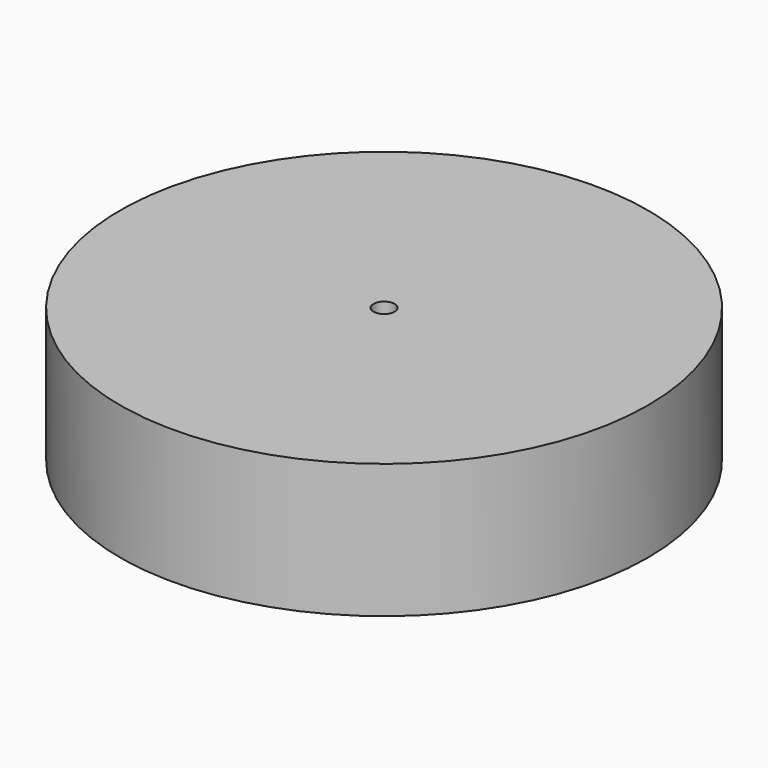
from build123d import *

# Parameters (mm, degrees)
F0_R     = 49.9999
F0_R_2   = 2.0066
F2_DEPTH = 25.4


# Not quite as in the source:
# - the program builds the solid bodies; features that only make, move or delete a surface that nothing else refers to are left out


with BuildPart() as f2:
    # F0 (on Top) → F2 (new body)
    with BuildSketch(Plane.XY):
        Circle(F0_R)
        Circle(F0_R_2, mode=Mode.SUBTRACT)
    extrude(amount=F2_DEPTH)


solid = f2.part
